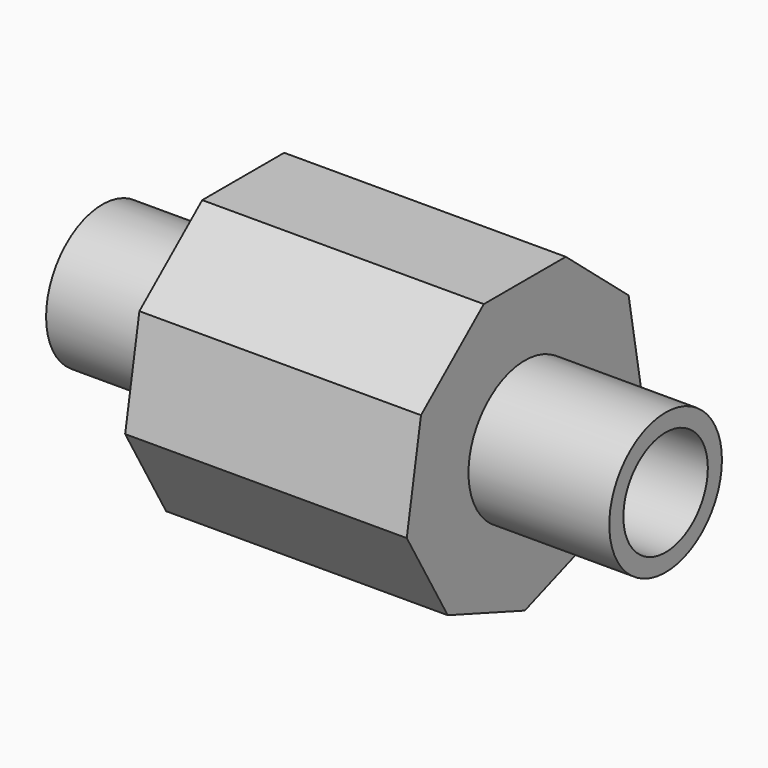
from build123d import *
from build123d import SkipClean  # not in build123d's __all__

# Parameters (mm, degrees)
F1_DEPTH = 50.8
F2_R     = 12.7
F3_DEPTH = 25.4
F4_R     = 9.525
F5_DEPTH = 76.2
F6_R     = 12.7
F6_R_2   = 9.525
F7_DEPTH = 25.4


with BuildPart() as f1:
    # F0 (on Right) → F1 (new body)
    with BuildSketch(Plane.YZ):
        Polygon((9.2448439504, 25.4), (-9.2448439504, 25.4), (-23.4087666217, 13.5150577104), (-26.6194672313, -4.693730285), (-17.3746232809, -20.706269715), (0, -27.0301154209), (17.3746232809, -20.706269715), (26.6194672313, -4.693730285), (23.4087666217, 13.5150577104), align=None)
    extrude(amount=F1_DEPTH)

    # F2 (on face) → F3 (join)
    with BuildSketch(Plane.YZ.offset(50.8)):
        Circle(F2_R)
    extrude(amount=F3_DEPTH)

    # F4 (on face) → F5 (cut)
    with BuildSketch(Plane.YZ.offset(76.2)):
        Circle(F4_R)
    extrude(amount=-F5_DEPTH, mode=Mode.SUBTRACT)

    # F6 (on face) → F7 (join)
    with BuildSketch(Plane(origin=(0, 0, 0), x_dir=(0, -1, 0), z_dir=(-1, 0, 0))):
        Circle(F6_R)
        Circle(F6_R_2, mode=Mode.SUBTRACT)
    with SkipClean():  # cleaning this boolean's faces spoils the solid; the shape is the same uncleaned
        extrude(amount=F7_DEPTH)


solid = f1.part
